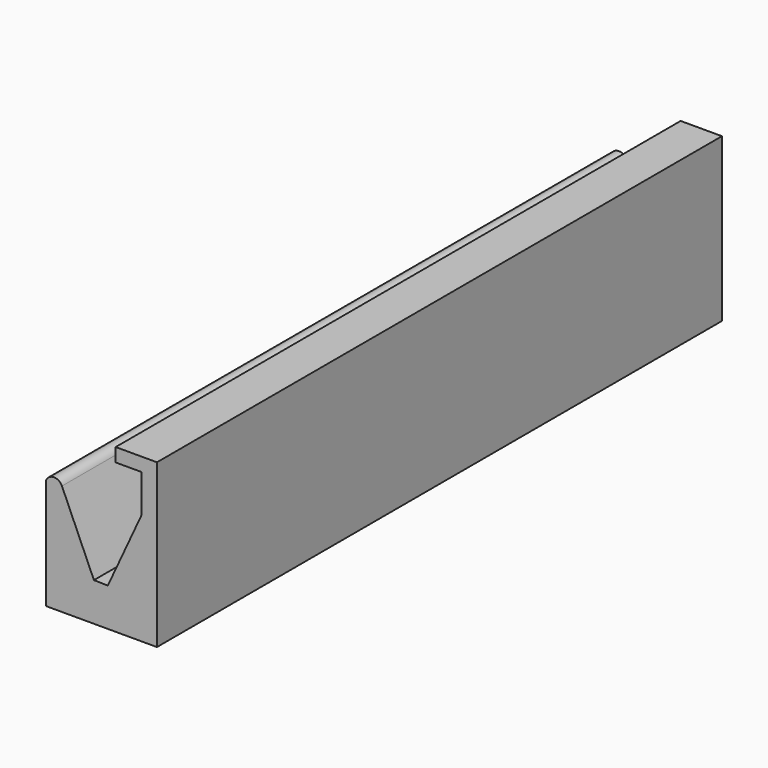
from build123d import *

# Parameters (mm, degrees)
F1_DEPTH = 25.4


# Not quite as in the source:
# - a feature names something its author has since deleted; it is built from what else it names


with BuildPart() as f1:
    # F0 (on Front) → F1 (new body)
    with BuildSketch(Plane.XZ):
        with BuildLine():
            Line((-1.9275679621, -0.9906), (2.0602320379, -0.9906))
            Line((2.0602320379, -0.9906), (2.0602320379, 2.9972))
            ThreePointArc((2.0602320379, 2.9972), (1.7808320379, 3.1758966119), (1.5014320379, 2.9972))
            Line((1.5014320379, 2.9972), (0.2927852911, 0.381))
            Line((0.2927852911, 0.381), (-0.2070155831, 0.3918310395))
            Line((-0.2070155831, 0.3918310395), (-1.3567524399, 2.9972))
            ThreePointArc((-1.3567524399, 2.9972), (-1.642160201, 3.1832136759), (-1.9275679621, 2.9972))
            Line((-1.9275679621, 2.9972), (-1.9275679621, -0.9906))
        make_face()
        with BuildLine():
            ThreePointArc((1.5014320379, 2.9972), (1.7808320379, 3.1758966119), (2.0602320379, 2.9972))
            Line((2.0602320379, 2.9972), (2.0602320379, 4.8607838479))
            Line((2.0602320379, 4.8607838479), (0.575090351, 4.8607838479))
            Line((0.575090351, 4.8607838479), (0.575090351, 4.3721500923))
            Line((0.575090351, 4.3721500923), (1.5014320379, 4.3721500923))
            Line((1.5014320379, 4.3721500923), (1.5014320379, 2.9972))
        make_face()
    extrude(amount=F1_DEPTH)


solid = f1.part
